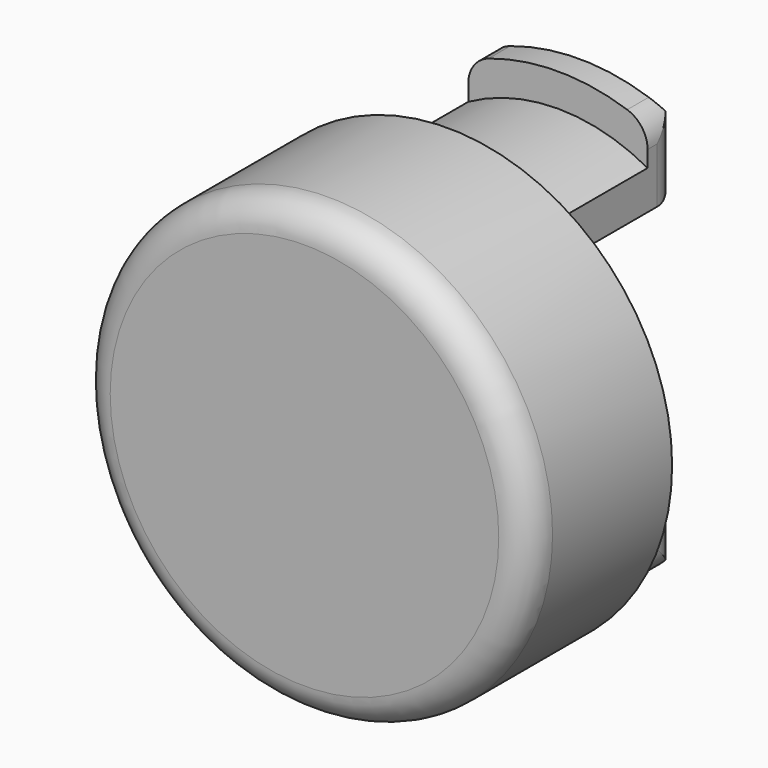
from build123d import *

# Parameters (mm, degrees)
F1_R         = 7.5
F2_DEPTH     = 6
F3_R         = 1
F4_T         = -2.4
F7_DEPTH     = 4.6
F9_DEPTH     = 1.4
F10_SIZE     = 0.5
F11_T1_DEPTH = 4.5650872514
F11_T3_DEPTH = 6.9781403955
F11_T5_DEPTH = 6.9781403955


# Not quite as in the source:
# - a fillet or chamfer that OpenCascade refuses, or shapes differently, is made with other operations: its cross-section is extruded or revolved along the edge and cut away or added


with BuildPart() as f2:
    # F1 (on offset) → F2 (new body)
    with BuildSketch(Plane.XZ.offset(13)):
        with Locations((-13, 13)):
            Circle(F1_R)
    extrude(amount=-F2_DEPTH)

    # F3
    f3_edges = [f2.edges().sort_by_distance(p)[0] for p in [
        (-20.5, -13, 13),
    ]]
    fillet(f3_edges, radius=F3_R)

    # F4
    f4_openings = [f2.faces().sort_by_distance(p)[0] for p in [
        (-13, -7, 13),
    ]]
    offset(amount=F4_T, openings=f4_openings)

    # F6 (on offset) → F7 (join, through all)
    with BuildSketch(Plane.XZ.offset(2.4)):
        with BuildLine():
            Line((-10, 17.1243181255), (-10, 18.4258639865))
            ThreePointArc((-10, 18.4258639865), (-13, 19.2), (-16, 18.4258639865))
            Line((-16, 18.4258639865), (-16, 17.1243181255))
            ThreePointArc((-16, 17.1243181255), (-13, 18.1), (-10, 17.1243181255))
        make_face()
        with BuildLine():
            ThreePointArc((-10, 8.8756818745), (-13, 7.9), (-16, 8.8756818745))
            Line((-16, 8.8756818745), (-16, 7.5741360135))
            ThreePointArc((-16, 7.5741360135), (-13, 6.8), (-10, 7.5741360135))
            Line((-10, 7.5741360135), (-10, 8.8756818745))
        make_face()
    extrude(amount=F7_DEPTH)

    # F8 (on offset) → F9 (join)
    with BuildSketch(Plane.XZ.offset(2.4)):
        with BuildLine():
            Line((-16, 8.8756818745), (-16, 6.3449267472))
            ThreePointArc((-16, 6.3449267472), (-13, 5.7), (-10, 6.3449267472))
            Line((-10, 6.3449267472), (-10, 8.8756818745))
            ThreePointArc((-10, 8.8756818745), (-13, 7.9), (-16, 8.8756818745))
        make_face()
        with BuildLine():
            Line((-10, 17.1243181255), (-10, 19.6550732528))
            ThreePointArc((-10, 19.6550732528), (-13, 20.3), (-16, 19.6550732528))
            Line((-16, 19.6550732528), (-16, 17.1243181255))
            ThreePointArc((-16, 17.1243181255), (-13, 18.1), (-10, 17.1243181255))
        make_face()
    extrude(amount=-F9_DEPTH)

    # F10
    f10_edges = [f2.edges().sort_by_distance(p)[0] for p in [
        (-13, -1, 5.7),
        (-13, -1, 20.3),
    ]]
    chamfer(f10_edges, length=F10_SIZE)

    # F11: fillet of radius 1 on 8 edges, made by hand

    # F11_s2 → F11_t1 (cut)
    with BuildSketch(Plane.XZ.offset(-0.3325436257)):
        with BuildLine():
            ThreePointArc((-10, 18.9741108125), (-10.1883780691, 19.5582938671), (-10.6825396825, 19.92238237))
            ThreePointArc((-10.6825396825, 19.92238237), (-10.3379125488, 19.7973002289), (-10, 19.6550732528))
            Line((-10, 19.6550732528), (-10, 18.9741108125))
        make_face()
        with BuildLine():
            ThreePointArc((-15.3174603175, 19.92238237), (-15.8116219309, 19.5582938671), (-16, 18.9741108125))
            Line((-16, 18.9741108125), (-16, 19.6550732528))
            ThreePointArc((-16, 19.6550732528), (-15.6620874512, 19.7973002289), (-15.3174603175, 19.92238237))
        make_face()
        with BuildLine():
            ThreePointArc((-10, 7.0258891875), (-10.1883780691, 6.4417061329), (-10.6825396825, 6.07761763))
            ThreePointArc((-10.6825396825, 6.07761763), (-10.3379125488, 6.2026997711), (-10, 6.3449267472))
            Line((-10, 6.3449267472), (-10, 7.0258891875))
        make_face()
        with BuildLine():
            ThreePointArc((-16, 7.0258891875), (-15.8116219309, 6.4417061329), (-15.3174603175, 6.07761763))
            ThreePointArc((-15.3174603175, 6.07761763), (-15.6620874512, 6.2026997711), (-16, 6.3449267472))
            Line((-16, 6.3449267472), (-16, 7.0258891875))
        make_face()
    extrude(amount=F11_T1_DEPTH, mode=Mode.SUBTRACT)

    # F11_s4 → F11_t3 (cut)
    with BuildSketch(Plane.XY.offset(14.6243181255)):
        with BuildLine():
            ThreePointArc((-10, -2), (-10.2928932188, -1.2928932188), (-11, -1))
            Line((-11, -1), (-10, -1))
            Line((-10, -1), (-10, -2))
        make_face()
        with BuildLine():
            ThreePointArc((-15, -1), (-15.7071067812, -1.2928932188), (-16, -2))
            Line((-16, -2), (-16, -1))
            Line((-16, -1), (-15, -1))
        make_face()
    extrude(amount=F11_T3_DEPTH, mode=Mode.SUBTRACT)

    # F11_s6 → F11_t5 (cut)
    with BuildSketch(Plane.XY.offset(4.397541479)):
        with BuildLine():
            ThreePointArc((-16, -2), (-15.7071067812, -1.2928932188), (-15, -1))
            Line((-15, -1), (-16, -1))
            Line((-16, -1), (-16, -2))
        make_face()
        with BuildLine():
            ThreePointArc((-10, -2), (-10.2928932188, -1.2928932188), (-11, -1))
            Line((-11, -1), (-10, -1))
            Line((-10, -1), (-10, -2))
        make_face()
    extrude(amount=F11_T5_DEPTH, mode=Mode.SUBTRACT)


solid = f2.part
